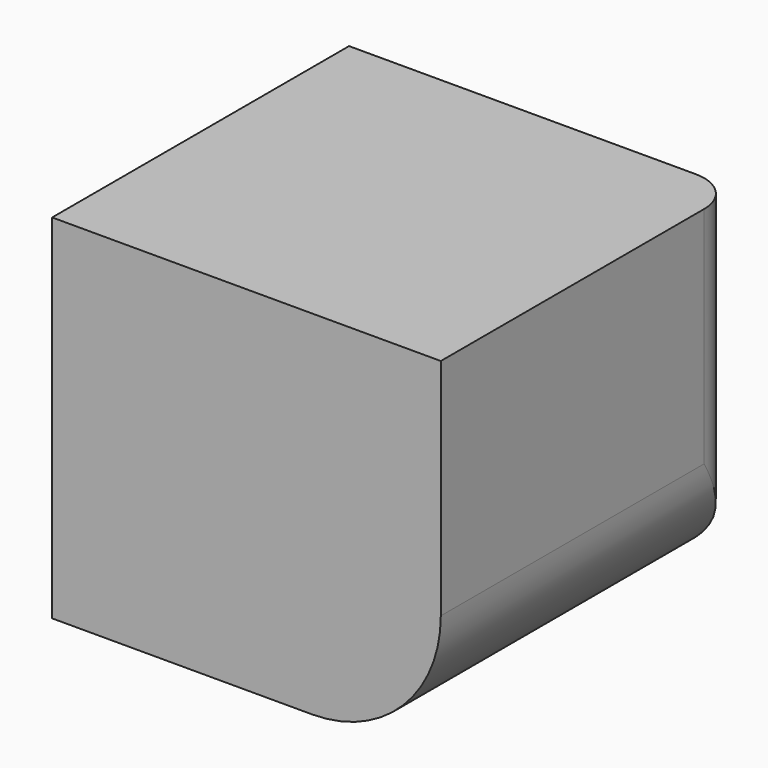
from build123d import *

# Parameters (mm, degrees)
F1_DEPTH    = 44.958
F2_T1_DEPTH = 52.5754828874


# Not quite as in the source:
# - a fillet or chamfer that OpenCascade refuses, or shapes differently, is made with other operations: its cross-section is extruded or revolved along the edge and cut away or added


with BuildPart() as f1:
    # F0 (on Front) → F1 (new body)
    with BuildSketch(Plane.XZ):
        with BuildLine():
            Line((35.7939489186, 14.252791281), (-11.2892372768, 14.252791281))
            Line((-11.2892372768, 14.252791281), (-11.2892372768, -28.5055878506))
            Line((-11.2892372768, -28.5055878506), (20.2110526745, -28.5055878506))
            ThreePointArc((20.2110526745, -28.5055878506), (31.2298242792, -23.9414632112), (35.7939489186, -12.9226916064))
            Line((35.7939489186, -12.9226916064), (35.7939489186, 14.252791281))
        make_face()
    extrude(amount=F1_DEPTH)

    # F2: fillet of radius 5.08 on 1 edges, made by hand

    # F2_s2 → F2_t1 (cut)
    with BuildSketch(Plane.XY.offset(-25.6226916064)):
        with BuildLine():
            ThreePointArc((35.7939489186, -5.08), (34.306051367, -1.4878975516), (30.7139489186, 0))
            Line((30.7139489186, 0), (35.7939489186, 0))
            Line((35.7939489186, 0), (35.7939489186, -5.08))
        make_face()
    extrude(amount=F2_T1_DEPTH, mode=Mode.SUBTRACT)


solid = f1.part
